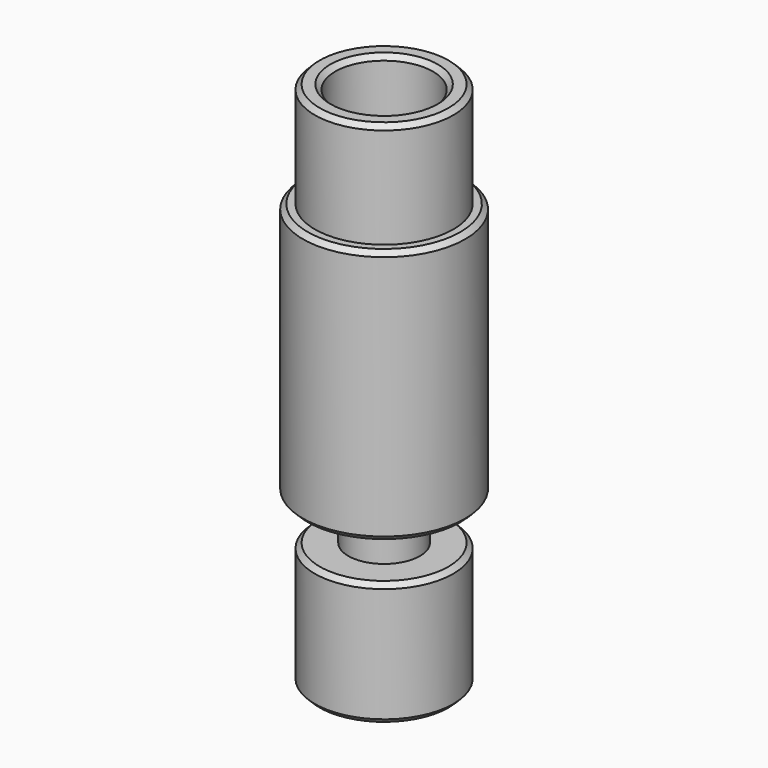
from build123d import *

# Parameters (mm, degrees)
F0_R     = 2.9
F0_R_2   = 1.5
F1_DEPTH = 22.11
F2_START = 7
F0_R_3   = 3.4
F2_DEPTH = 10.7
F3_START = 5.2
F3_DEPTH = 1.8
F5_D     = 2.1
F6_D     = 4.1
F6_DEPTH = 4.4
F6_TIP   = 1.231764269
F7_SIZE  = 0.2


with BuildPart() as f1:
    # F0 (on Top) → F1 (new body)
    with BuildSketch(Plane.XY):
        Circle(F0_R)
        Circle(F0_R_2, mode=Mode.SUBTRACT)
        Circle(F0_R_2)
    extrude(amount=F1_DEPTH)

    # F0 (on Top) → F2 (join)
    with BuildSketch(Plane.XY.offset(F2_START)):
        Circle(F0_R_3)
        Circle(F0_R, mode=Mode.SUBTRACT)
    extrude(amount=F2_DEPTH)

    # F0 (on Top) → F3 (cut)
    with BuildSketch(Plane.XY.offset(F3_START)):
        Circle(F0_R_3)
        Circle(F0_R, mode=Mode.SUBTRACT)
        Circle(F0_R)
        Circle(F0_R_2, mode=Mode.SUBTRACT)
    extrude(amount=F3_DEPTH, mode=Mode.SUBTRACT)

    # F5 (through all)
    with Locations(Plane.XY.offset(22.11)):
        with Locations((0, 0)):
            Hole(F5_D / 2)

    # F6
    with Locations(Plane.XY.offset(22.11)):
        with Locations((0, 0)):
            Hole(F6_D / 2, depth=F6_DEPTH)
            with Locations((0, 0, -(F6_DEPTH + F6_TIP / 2))):  # 118° drill point
                Cone(0, F6_D / 2, F6_TIP, mode=Mode.SUBTRACT)

    # F7
    f7_edges = [f1.edges().sort_by_distance(p)[0] for p in [
        (-2.9, 0, 22.11),
        (-2.9, 0, 5.2),
        (-2.9, 0, 0),
        (-3.4, 0, 7),
        (-3.4, 0, 17.7),
        (-2.05, 0, 22.11),
    ]]
    chamfer(f7_edges, length=F7_SIZE)


solid = f1.part
